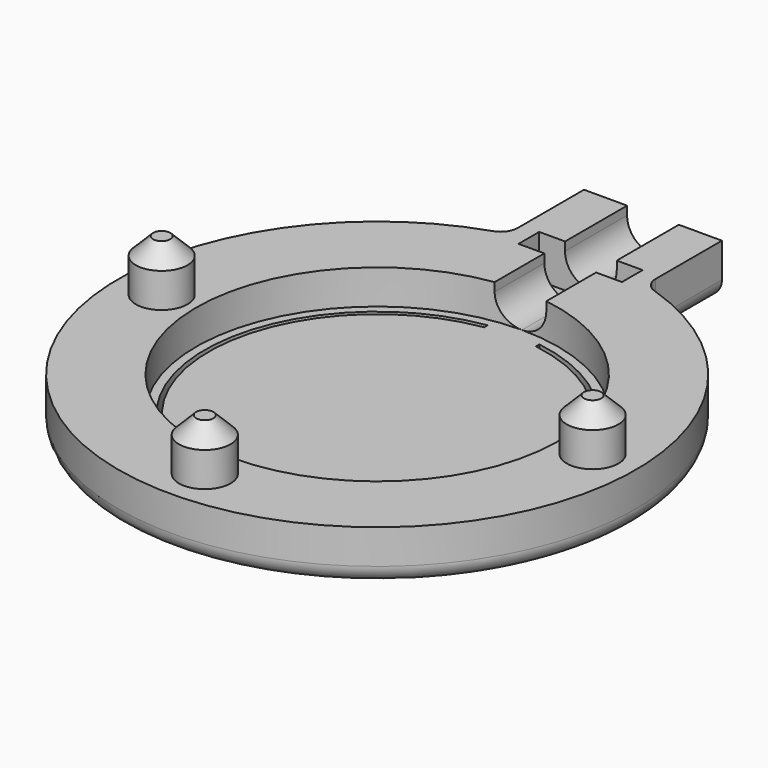
from build123d import *

# Parameters (mm, degrees)
F1_DEPTH  = 3
F3_DEPTH  = 2
F4_R      = 1.5
F5_DEPTH  = 3
F6_SIZE   = 1
F7_R      = 1
F9_DEPTH  = 1.0010001
F10_R     = 1.49999
F11_W     = 6
F11_H     = 1.5
F12_DEPTH = 2.5


# Not quite as in the source:
# - a fillet or chamfer is up to 0.001 mm smaller than in the source, because OpenCascade refuses the exact size


with BuildPart() as f1:
    # F0 (on Top) → F1 (new body)
    with BuildSketch(Plane.XY):
        with BuildLine():
            Line((-4, 20), (-4, 14.4568322948))
            ThreePointArc((-4, 14.4568322948), (0, -15), (4, 14.4568322948))
            Line((4, 14.4568322948), (4, 20))
            Line((4, 20), (-4, 20))
        make_face()
    extrude(amount=F1_DEPTH)

    # F2 (on face) → F3 (cut)
    with BuildSketch(Plane.XY.offset(3)):
        with BuildLine():
            Line((1.5, 20), (-1.5, 20))
            Line((-1.5, 20), (-1.5, 10.3923048454))
            ThreePointArc((-1.5, 10.3923048454), (0, -10.5), (1.5, 10.3923048454))
            Line((1.5, 10.3923048454), (1.5, 20))
        make_face()
    extrude(amount=-F3_DEPTH, mode=Mode.SUBTRACT)

    # F4 (on face) → F5 (join)
    with BuildSketch(Plane.XY.offset(3)):
        with Locations((12.5, 0)):
            Circle(F4_R)
        with Locations((-12.5, 0)):
            Circle(F4_R)
        with Locations((0, -12.5)):
            Circle(F4_R)
    extrude(amount=F5_DEPTH)

    # F6
    f6_edges = [f1.edges().sort_by_distance(p)[0] for p in [
        (-14, 0, 6),
        (-1.5, -12.5, 6),
        (11, 0, 6),
    ]]
    chamfer(f6_edges, length=F6_SIZE)

    # F7
    f7_edges = [f1.edges().sort_by_distance(p)[0] for p in [
        (4, 17.228416, 0),
        (4, 14.456832, 1.5),
        (-4, 14.456832, 1.5),
        (-4, 17.228416, 0),
        (0, -15, 0),
    ]]
    fillet(f7_edges, radius=F7_R)

    # F8 (on face) → F9 (cut, through all)
    with BuildSketch(Plane.XY.offset(1)):
        with BuildLine():
            Line((-1.5, 9.633924434), (-1.5, 9.8868599666))
            ThreePointArc((-1.5, 9.8868599666), (0, -10), (1.5, 9.8868599666))
            Line((1.5, 9.8868599666), (1.5, 9.633924434))
            ThreePointArc((1.5, 9.633924434), (0, -9.75), (-1.5, 9.633924434))
        make_face()
    extrude(amount=-F9_DEPTH, mode=Mode.SUBTRACT)

    # F10 (radius 1.5 in the source; OpenCascade refuses exactly that, so slightly less here)
    f10_edges = [f1.edges().sort_by_distance(p)[0] for p in [
        (1.5, 15.196152, 1),
        (-1.5, 15.196152, 1),
    ]]
    fillet(f10_edges, radius=F10_R)

    # F11 (on face) → F12 (cut)
    with BuildSketch(Plane.XY.offset(3)):
        with Locations((0, 14.75)):
            Rectangle(F11_W, F11_H)
    extrude(amount=-F12_DEPTH, mode=Mode.SUBTRACT)


solid = f1.part
